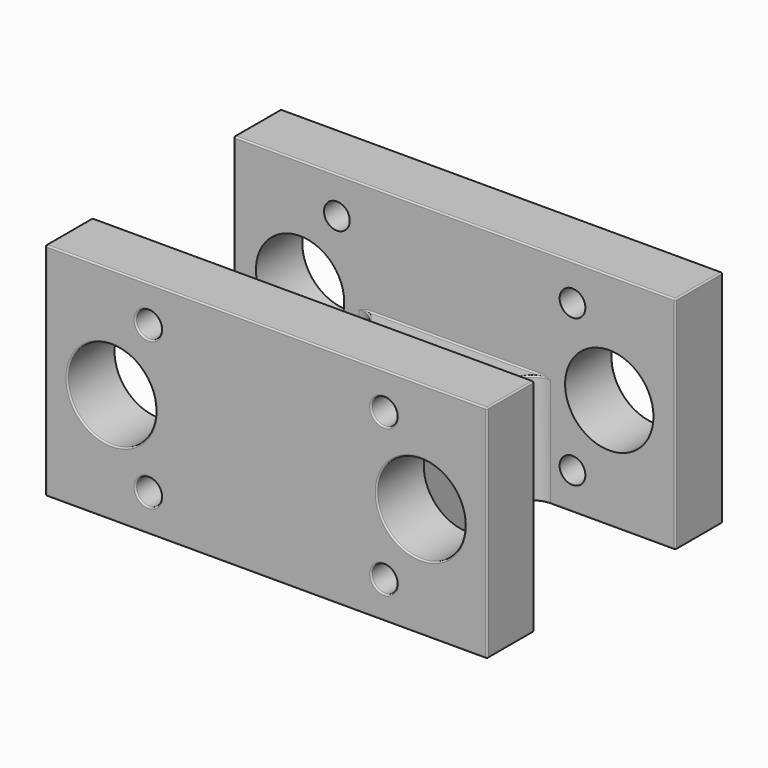
from build123d import *

# Parameters (mm, degrees)
F0_W      = 60
F0_H      = 40
F0_R      = 6
F1_DEPTH  = 7.5
F2_W      = 8
F2_H      = 15
F3_DEPTH  = 60
F4_R      = 1.75
F5_DEPTH  = 8
F6_R      = 1.75
F7_DEPTH  = 8
F8_R      = 7.5
F9_DEPTH  = 0.8
F10_R     = 7.5
F11_DEPTH = 0.8
F12_W     = 20
F12_H     = 24
F13_DEPTH = 25
F14_R     = 3
F15_R     = 6
F16_DEPTH = 40.001
F17_F1_R  = 0.2
F17_F2_R  = 0.2
F17_F3_R  = 0.2
F17_F4_R  = 0.2
F17_F5_R  = 0.2
F17_F6_R  = 0.2
F17_F7_R  = 0.2
F17_F8_R  = 0.2
F17_F9_R  = 0.2
F17_F10_R = 0.2
F17_F11_R = 0.2
F17_F12_R = 0.2
F17_F13_R = 0.2
F17_F14_R = 0.2
F17_F15_R = 0.2
F17_F16_R = 0.2
F17_F17_R = 0.2
F17_F18_R = 0.2
F17_F19_R = 0.2
F17_F20_R = 0.2
F17_F21_R = 0.2
F17_F22_R = 0.2
F17_F23_R = 0.2
F17_F24_R = 0.2
F17_F25_R = 0.2
F17_F26_R = 0.2
F17_F27_R = 0.2
F17_F28_R = 0.2
F17_F29_R = 0.2
F17_F30_R = 0.2


with BuildPart() as f1:
    # F0 (on Top) → F1 (new body, symmetric)
    with BuildSketch(Plane.XY):
        Rectangle(F0_W, F0_H)
        Circle(F0_R, mode=Mode.SUBTRACT)
    extrude(amount=F1_DEPTH, both=True)

    # F2 (on face) → F3 (join, through all)
    with BuildSketch(Plane.YZ.offset(30)):
        with Locations((16, 15)):
            Rectangle(F2_W, F2_H)
        with Locations((-16, 15)):
            Rectangle(F2_W, F2_H)
    extrude(amount=-F3_DEPTH)

    # F4 (on face) → F5 (cut)
    with BuildSketch(Plane(origin=(0, 20, 0), x_dir=(-1, 0, 0), z_dir=(0, 1, 0))):
        with Locations((16, 17.5)):
            Circle(F4_R)
        with Locations((-16, 17.5)):
            Circle(F4_R)
        with Locations((16, -2.5)):
            Circle(F4_R)
        with Locations((-16, -2.5)):
            Circle(F4_R)
    extrude(amount=-F5_DEPTH, mode=Mode.SUBTRACT)

    # F6 (on face) → F7 (cut)
    with BuildSketch(Plane.XZ.offset(20)):
        with Locations((16, 17.5)):
            Circle(F6_R)
        with Locations((-16, 17.5)):
            Circle(F6_R)
        with Locations((16, -2.5)):
            Circle(F6_R)
        with Locations((-16, -2.5)):
            Circle(F6_R)
    extrude(amount=-F7_DEPTH, mode=Mode.SUBTRACT)

    # F8 (on face) → F9 (cut)
    with BuildSketch(Plane.XY.offset(7.5)):
        Circle(F8_R)
    extrude(amount=-F9_DEPTH, mode=Mode.SUBTRACT)

    # F10 (on face) → F11 (cut)
    with BuildSketch(Plane(origin=(0, 0, -7.5), x_dir=(1, 0, 0), z_dir=(0, 0, -1))):
        Circle(F10_R)
    extrude(amount=-F11_DEPTH, mode=Mode.SUBTRACT)

    # F12 (on face) → F13 (cut)
    with BuildSketch(Plane.XY.offset(7.5)):
        with Locations((20, 0)):
            Rectangle(F12_W, F12_H)
        with Locations((-20, 0)):
            Rectangle(F12_W, F12_H)
    extrude(amount=-F13_DEPTH, mode=Mode.SUBTRACT)

    # F14
    f14_edges = [f1.edges().sort_by_distance(p)[0] for p in [
        (-10, 12, 0),
        (-10, -12, 0),
        (10, 12, 0),
        (10, -12, 0),
    ]]
    fillet(f14_edges, radius=F14_R)

    # F15 (on face) → F16 (cut, through all)
    with BuildSketch(Plane.XZ.offset(20)):
        with Locations((-21, 7.5)):
            Circle(F15_R)
        with Locations((21, 7.5)):
            Circle(F15_R)
    extrude(amount=-F16_DEPTH, mode=Mode.SUBTRACT)

    # F17: fillet of radius 0.2 on 54 edges, made by hand

    # F17_f1
    f17_f1_edges = [f1.edges().sort_by_distance(p)[0] for p in [
        (21.5, -12, -7.5),
        (10.8786796564, -11.1213203436, -7.5),
        (10, 0, -7.5),
        (10.8786796564, 11.1213203436, -7.5),
        (21.5, 12, -7.5),
    ]]
    fillet(f17_f1_edges, radius=F17_F1_R)

    # F17_f2
    f17_f2_edges = [f1.edges().sort_by_distance(p)[0] for p in [
        (-21.5, -12, -7.5),
        (-21.5, 12, -7.5),
        (-10.8786796564, 11.1213203436, -7.5),
        (-10, 0, -7.5),
        (-10.8786796564, -11.1213203436, -7.5),
    ]]
    fillet(f17_f2_edges, radius=F17_F2_R)

    # F17_f3
    f17_f3_edges = [f1.edges().sort_by_distance(p)[0] for p in [
        (0, -12, 22.5),
    ]]
    fillet(f17_f3_edges, radius=F17_F3_R)

    # F17_f4
    f17_f4_edges = [f1.edges().sort_by_distance(p)[0] for p in [
        (0, -20, -7.5),
    ]]
    fillet(f17_f4_edges, radius=F17_F4_R)

    # F17_f5
    f17_f5_edges = [f1.edges().sort_by_distance(p)[0] for p in [
        (0, -20, 22.5),
    ]]
    fillet(f17_f5_edges, radius=F17_F5_R)

    # F17_f6
    f17_f6_edges = [f1.edges().sort_by_distance(p)[0] for p in [
        (0, 12, 22.5),
    ]]
    fillet(f17_f6_edges, radius=F17_F6_R)

    # F17_f7
    f17_f7_edges = [f1.edges().sort_by_distance(p)[0] for p in [
        (0, 20, -7.5),
    ]]
    fillet(f17_f7_edges, radius=F17_F7_R)

    # F17_f8
    f17_f8_edges = [f1.edges().sort_by_distance(p)[0] for p in [
        (0, 20, 22.5),
    ]]
    fillet(f17_f8_edges, radius=F17_F8_R)

    # F17_f9
    f17_f9_edges = [f1.edges().sort_by_distance(p)[0] for p in [
        (-7.5, 0, 7.5),
    ]]
    fillet(f17_f9_edges, radius=F17_F9_R)

    # F17_f10
    f17_f10_edges = [f1.edges().sort_by_distance(p)[0] for p in [
        (-7.5, 0, -7.5),
    ]]
    fillet(f17_f10_edges, radius=F17_F10_R)

    # F17_f11
    f17_f11_edges = [f1.edges().sort_by_distance(p)[0] for p in [
        (15, -20, 7.5),
    ]]
    fillet(f17_f11_edges, radius=F17_F11_R)

    # F17_f12
    f17_f12_edges = [f1.edges().sort_by_distance(p)[0] for p in [
        (15, 20, 7.5),
    ]]
    fillet(f17_f12_edges, radius=F17_F12_R)

    # F17_f13
    f17_f13_edges = [f1.edges().sort_by_distance(p)[0] for p in [
        (-27, 20, 7.5),
    ]]
    fillet(f17_f13_edges, radius=F17_F13_R)

    # F17_f14
    f17_f14_edges = [f1.edges().sort_by_distance(p)[0] for p in [
        (-27, -20, 7.5),
    ]]
    fillet(f17_f14_edges, radius=F17_F14_R)

    # F17_f15
    f17_f15_edges = [f1.edges().sort_by_distance(p)[0] for p in [
        (30, -12, 7.5),
    ]]
    fillet(f17_f15_edges, radius=F17_F15_R)

    # F17_f16
    f17_f16_edges = [f1.edges().sort_by_distance(p)[0] for p in [
        (-30, -12, 7.5),
    ]]
    fillet(f17_f16_edges, radius=F17_F16_R)

    # F17_f17
    f17_f17_edges = [f1.edges().sort_by_distance(p)[0] for p in [
        (-30, 12, 7.5),
    ]]
    fillet(f17_f17_edges, radius=F17_F17_R)

    # F17_f18
    f17_f18_edges = [f1.edges().sort_by_distance(p)[0] for p in [
        (30, 12, 7.5),
    ]]
    fillet(f17_f18_edges, radius=F17_F18_R)

    # F17_f19
    f17_f19_edges = [f1.edges().sort_by_distance(p)[0] for p in [
        (10.8786796564, -11.1213203436, 7.5),
        (10, 0, 7.5),
        (10.8786796564, 11.1213203436, 7.5),
    ]]
    fillet(f17_f19_edges, radius=F17_F19_R)

    # F17_f20
    f17_f20_edges = [f1.edges().sort_by_distance(p)[0] for p in [
        (-10.8786796564, 11.1213203436, 7.5),
        (-10, 0, 7.5),
        (-10.8786796564, -11.1213203436, 7.5),
    ]]
    fillet(f17_f20_edges, radius=F17_F20_R)

    # F17_f21
    f17_f21_edges = [f1.edges().sort_by_distance(p)[0] for p in [
        (0, -12, 7.5),
    ]]
    fillet(f17_f21_edges, radius=F17_F21_R)

    # F17_f22
    f17_f22_edges = [f1.edges().sort_by_distance(p)[0] for p in [
        (0, 12, 7.5),
    ]]
    fillet(f17_f22_edges, radius=F17_F22_R)

    # F17_f23
    f17_f23_edges = [f1.edges().sort_by_distance(p)[0] for p in [
        (14.25, -20, 17.5),
    ]]
    fillet(f17_f23_edges, radius=F17_F23_R)

    # F17_f24
    f17_f24_edges = [f1.edges().sort_by_distance(p)[0] for p in [
        (14.25, -20, -2.5),
    ]]
    fillet(f17_f24_edges, radius=F17_F24_R)

    # F17_f25
    f17_f25_edges = [f1.edges().sort_by_distance(p)[0] for p in [
        (-14.25, 20, 17.5),
    ]]
    fillet(f17_f25_edges, radius=F17_F25_R)

    # F17_f26
    f17_f26_edges = [f1.edges().sort_by_distance(p)[0] for p in [
        (-14.25, 20, -2.5),
    ]]
    fillet(f17_f26_edges, radius=F17_F26_R)

    # F17_f27
    f17_f27_edges = [f1.edges().sort_by_distance(p)[0] for p in [
        (-17.75, -20, -2.5),
    ]]
    fillet(f17_f27_edges, radius=F17_F27_R)

    # F17_f28
    f17_f28_edges = [f1.edges().sort_by_distance(p)[0] for p in [
        (-17.75, -20, 17.5),
    ]]
    fillet(f17_f28_edges, radius=F17_F28_R)

    # F17_f29
    f17_f29_edges = [f1.edges().sort_by_distance(p)[0] for p in [
        (17.75, 20, -2.5),
    ]]
    fillet(f17_f29_edges, radius=F17_F29_R)

    # F17_f30
    f17_f30_edges = [f1.edges().sort_by_distance(p)[0] for p in [
        (17.75, 20, 17.5),
    ]]
    fillet(f17_f30_edges, radius=F17_F30_R)


solid = f1.part
